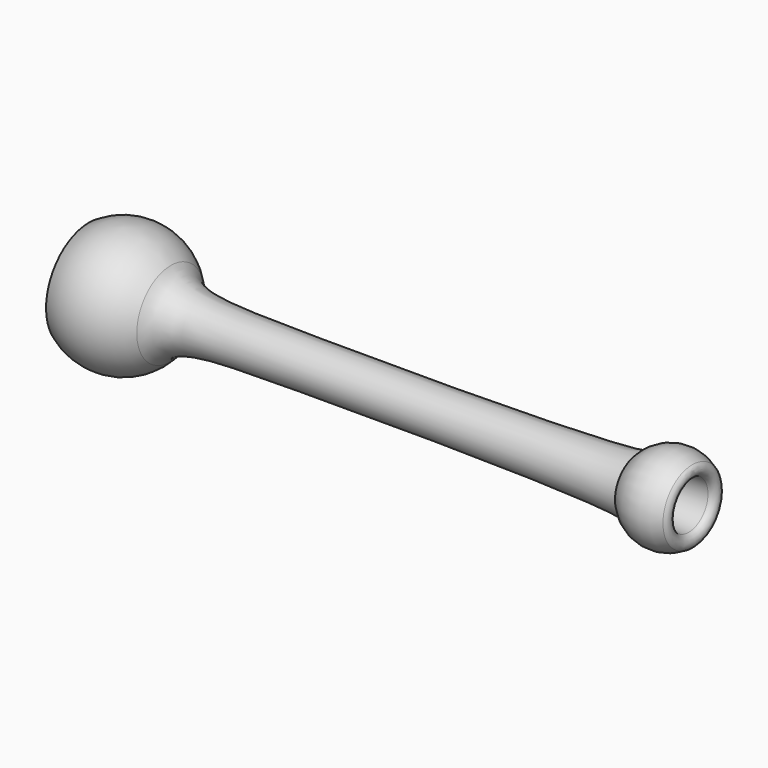
from build123d import *

# Parameters (mm, degrees)
F2_R = 2


# Not quite as in the source:
# - a fillet or chamfer that OpenCascade refuses, or shapes differently, is made with other operations: its cross-section is extruded or revolved along the edge and cut away or added


with BuildPart() as f1:
    # F0 (on Front) → F1 (revolve)
    with BuildSketch(Plane.XZ):
        with BuildLine():
            ThreePointArc((-7.0685046336, 10.3095219212), (4.6853520259, 11.5886788028), (12.2474487139, 2.5))
            Line((12.2474487139, 2.5), (74.2474487139, 2.5))
            Line((74.2474487139, 2.5), (168.7871957085, 7.1925999325))
            ThreePointArc((168.7871957085, 7.1925999325), (159.5167247738, 12.593006562), (149.6324140859, 8.4209057314))
            add(Edge.make_bspline(
                [(13.7809895682, 12.3177978136), (16.9480145501, 7.0949664659), (43.0290831579, 6.1845923366), (140.8783346117, 6.3666986814), (149.6324140859, 8.4209057314)],
                knots=[0, 0, 0, 0, 0.3508638512, 1, 1, 1, 1], degree=3))
            ThreePointArc((13.7809895682, 12.3177978136), (2.4835532955, 18.3159979112), (-10.003236638, 15.5428141988))
            Line((-10.003236638, 15.5428141988), (-7.0685046336, 10.3095219212))
        make_face()
    revolve(axis=Axis((35, 0, 0), (1, 0, 0)))

    # F2
    f2_edges = [f1.edges().sort_by_distance(p)[0] for p in [
        (168.787196, 0, -7.1926),
        (-7.068505, 0, -10.309522),
        (12.247449, 0, -2.5),
    ]]
    fillet(f2_edges, radius=F2_R)

    # F3: fillet of radius 5 on 1 edges, made by hand

    # F3_s1 → F3_t2 (revolve, cut)
    with BuildSketch(Plane.XZ):
        with BuildLine():
            ThreePointArc((74.371310549, 2.5061480389), (74.2474105858, 2.501537246), (74.1234343898, 2.5))
            Line((74.1234343898, 2.5), (74.1234343898, 2.4))
            Line((74.1234343898, 2.4), (74.2499290004, 2.4))
            Line((74.2499290004, 2.4), (74.3762680722, 2.4062709996))
            Line((74.3762680722, 2.4062709996), (74.371310549, 2.5061480389))
        make_face()
    revolve(axis=Axis((74.2474487139, 0, 0), (1, 0, 0)), mode=Mode.SUBTRACT)


solid = f1.part
